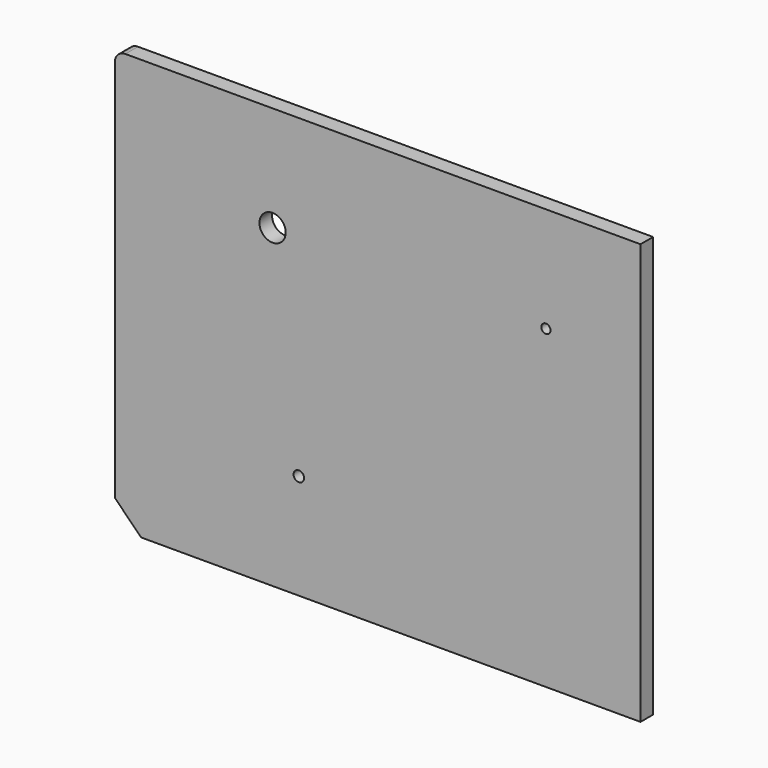
from build123d import *

# Parameters (mm, degrees)
F0_W     = 1000
F0_H     = 800
F1_DEPTH = 15
F3_D     = 50
F4_D     = 20
F5_D     = 17.5
F6_R     = 20
F7_SIZE  = 50


with BuildPart() as f1:
    # F0 (on Front) → F1 (new body, symmetric)
    with BuildSketch(Plane.XZ):
        Rectangle(F0_W, F0_H)
    extrude(amount=F1_DEPTH, both=True)

    # F3 (through all)
    with Locations(Plane.XZ.offset(15)):
        with Locations((-200, 200)):
            Hole(F3_D / 2)

    # F4 (through all)
    with Locations(Plane.XZ.offset(15)):
        with Locations((-150, -200)):
            Hole(F4_D / 2)

    # F5 (through all)
    with Locations(Plane.XZ.offset(15)):
        with Locations((320, 200)):
            Hole(F5_D / 2)

    # F6
    f6_edges = [f1.edges().sort_by_distance(p)[0] for p in [
        (-500, 0, 400),
    ]]
    fillet(f6_edges, radius=F6_R)

    # F7
    f7_edges = [f1.edges().sort_by_distance(p)[0] for p in [
        (-500, 0, -400),
    ]]
    chamfer(f7_edges, length=F7_SIZE)


solid = f1.part
